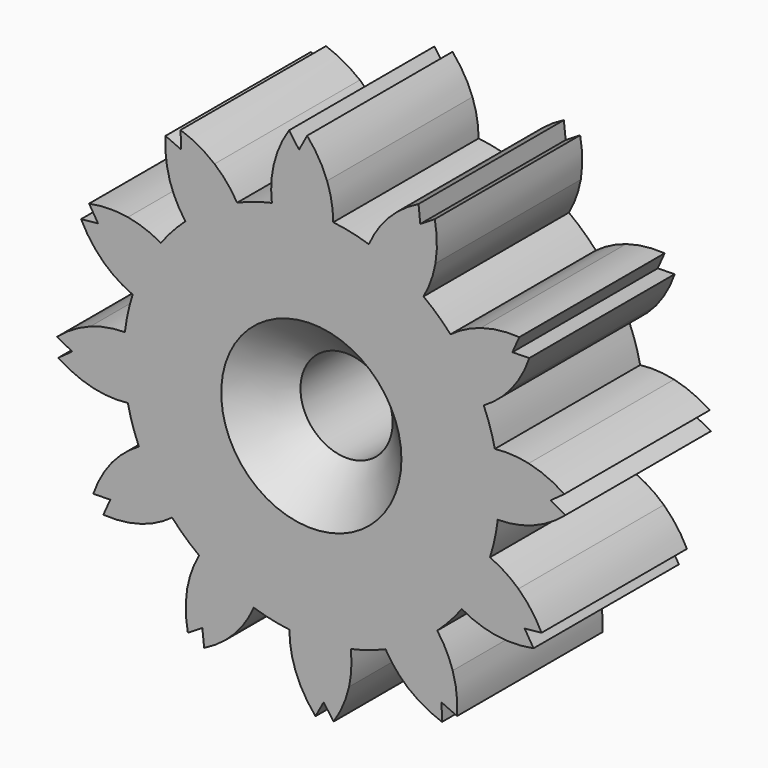
from build123d import *

# Parameters (mm, degrees)
F0_R     = 6.5928960908
F1_DEPTH = 26
F2_COUNT = 12
F3_SIZE  = 6.3


# Not quite as in the source:
# - a feature names something its author has since deleted; it is built from what else it names


with BuildPart() as f1:
    # F0 (on Front) → F1 (new body)
    with BuildSketch(Plane.XZ):
        with BuildLine():
            ThreePointArc((-5.6485408912, 26.2598637858), (-16.878445243, -20.8950842647), (26.8605, 0))
            ThreePointArc((26.8605, 0), (20.0726478905, 17.8486768953), (3.1397750014, 26.6763616933))
            ThreePointArc((3.1397750014, 26.6763616933), (-1.2715518862, 26.8303860585), (-5.6485408912, 26.2598637858))
        make_face()
        Circle(F0_R, mode=Mode.SUBTRACT)
        with BuildLine():
            ThreePointArc((-5.6485408912, 26.2598637858), (-1.2715518862, 26.8303860585), (3.1397750014, 26.6763616933))
            ThreePointArc((3.1397750014, 26.6763616933), (2.912439248, 29.1823081791), (2.258607373, 31.6121133592))
            ThreePointArc((2.258607373, 31.6121133592), (1.0476425624, 34.1233003108), (-0.5978331908, 36.3738347416))
            Line((-0.5978331908, 36.3738347416), (-1.7586341705, 34.2293752337))
            Line((-1.7586341705, 34.2293752337), (-3.1894124709, 36.2039736615))
            ThreePointArc((-3.1894124709, 36.2039736615), (-4.5270572612, 33.7579151802), (-5.3998864293, 31.1101491555))
            ThreePointArc((-5.3998864293, 31.1101491555), (-5.727107406, 28.6954080102), (-5.6485408912, 26.2598637858))
        make_face()
    extrude(amount=F1_DEPTH)

    # F2: F1 ×12 about axis
    f2_axis = Axis((0, 0, 0), (0, 1, 0))


with BuildPart() as f1_1:
    add(f1.part)
    for i in range(1, F2_COUNT):
        add(f1.part.rotate(f2_axis, i * 360 / F2_COUNT))

    # F3
    f3_edges = [f1_1.edges().sort_by_distance(p)[0] for p in [
        (-6.592896, 0, 0),
        (6.592896, -13, 0),
        (-6.592896, -26, 0),
    ]]
    chamfer(f3_edges, length=F3_SIZE)


solid = f1_1.part
